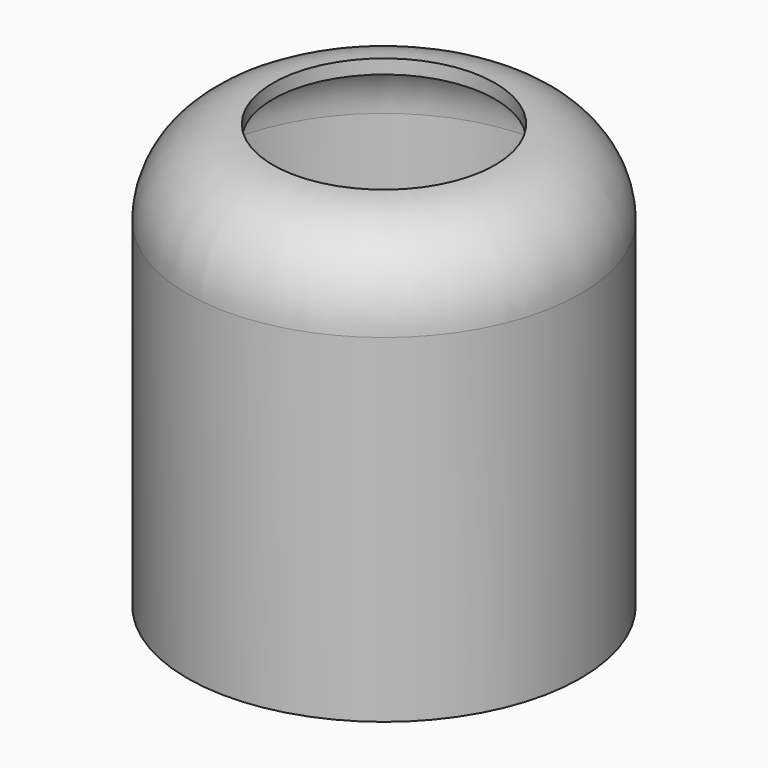
from build123d import *

# Parameters (mm, degrees)
F0_R     = 35.2243618103
F1_DEPTH = 75.946
F2_R     = 15.3302561211
F3_T     = -2.54


# Not quite as in the source:
# - a shell that OpenCascade refuses in one call is made with other operations: the cavity is built on its own and cut out


with BuildPart() as f1:
    # F0 (on Top) → F1 (new body)
    with BuildSketch(Plane.XY):
        with Locations((-4.9064448103, -47.139827162)):
            Circle(F0_R)
    extrude(amount=F1_DEPTH)

    # F2
    f2_edges = [f1.edges().sort_by_distance(p)[0] for p in [
        (-40.130807, -47.139827, 75.946),
    ]]
    fillet(f2_edges, radius=F2_R)

    # F3: a shell. OpenCascade refuses it in one call, so the cavity is built on its own and cut out:
    # the body offset inwards by the wall thickness, plus a prism from it out through each open face.
    f3_core = offset(f1.part, amount=F3_T, mode=Mode.PRIVATE)
    f3_exits = [f3_core.faces().sort_by_distance(p)[0] for p in [
        (-4.906445, -47.139827, 73.406),
    ]]
    add(f3_core, mode=Mode.SUBTRACT)
    extrude(f3_exits, amount=-F3_T, mode=Mode.SUBTRACT)


solid = f1.part
